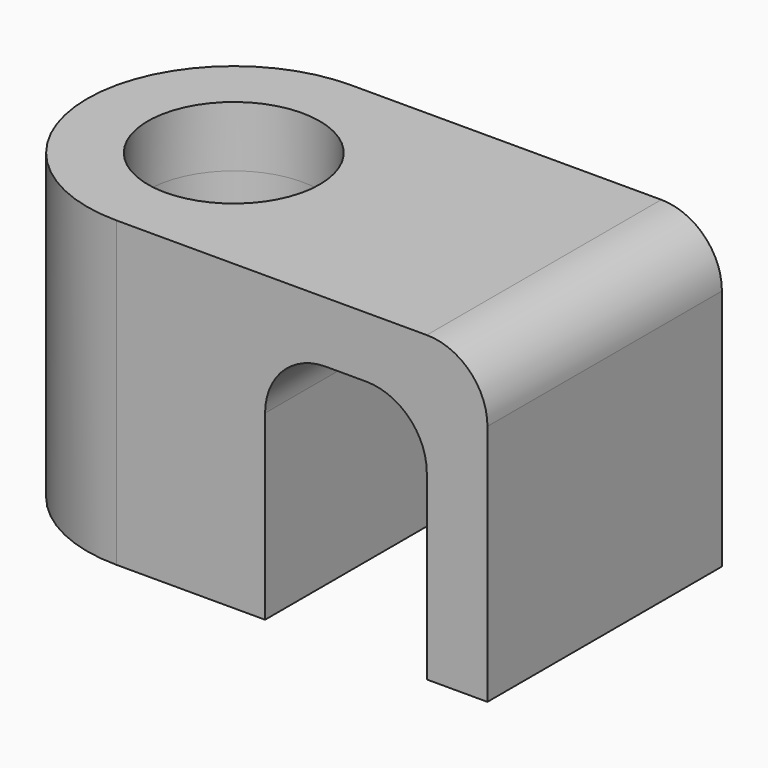
from build123d import *

# Parameters (mm, degrees)
F0_R        = 4.25
F0_W        = 8
F0_H        = 14.5
F0_W_2      = 3
F1_DEPTH    = 3
F2_DEPTH    = 12
F3_T1_DEPTH = 14.5
F3_T3_DEPTH = 29.5
F5_R        = 4.25
F6_DEPTH    = 22
F7_DEPTH    = 3
F8_T1_DEPTH = 28


# Not quite as in the source:
# - a fillet or chamfer that OpenCascade refuses, or shapes differently, is made with other operations: its cross-section is extruded or revolved along the edge and cut away or added


with BuildPart() as f1:
    # F0 (on Top) → F1 (new body)
    with BuildSketch(Plane.XY):
        with BuildLine():
            ThreePointArc((0, -7.25), (5.1265241636, -5.1265241636), (7.25, 0))
            ThreePointArc((7.25, 0), (5.1265241636, 5.1265241636), (0, 7.25))
            ThreePointArc((0, 7.25), (-7.25, 0), (0, -7.25))
        make_face()
        Circle(F0_R, mode=Mode.SUBTRACT)
        with BuildLine():
            Line((7.25, -7.25), (7.25, 0))
            ThreePointArc((7.25, 0), (5.1265241636, -5.1265241636), (0, -7.25))
            Line((0, -7.25), (7.25, -7.25))
        make_face()
        with BuildLine():
            ThreePointArc((0, 7.25), (5.1265241636, 5.1265241636), (7.25, 0))
            Line((7.25, 0), (7.25, 7.25))
            Line((7.25, 7.25), (0, 7.25))
        make_face()
        Polygon((7.25, 7.25), (7.25, 0), (7.25, -7.25), (7.35, -7.25), (7.35, 7.25), align=None)
        with Locations((11.35, 0)):
            Rectangle(F0_W, F0_H)
        with Locations((16.85, 0)):
            Rectangle(F0_W_2, F0_H)
    extrude(amount=F1_DEPTH)

    # F0 (on Top) → F2 (join)
    with BuildSketch(Plane.XY):
        with BuildLine():
            ThreePointArc((0, -7.25), (5.1265241636, -5.1265241636), (7.25, 0))
            ThreePointArc((7.25, 0), (5.1265241636, 5.1265241636), (0, 7.25))
            ThreePointArc((0, 7.25), (-7.25, 0), (0, -7.25))
        make_face()
        Circle(F0_R, mode=Mode.SUBTRACT)
        with BuildLine():
            ThreePointArc((0, 7.25), (5.1265241636, 5.1265241636), (7.25, 0))
            Line((7.25, 0), (7.25, 7.25))
            Line((7.25, 7.25), (0, 7.25))
        make_face()
        Polygon((7.25, 7.25), (7.25, 0), (7.25, -7.25), (7.35, -7.25), (7.35, 7.25), align=None)
        with Locations((16.85, 0)):
            Rectangle(F0_W_2, F0_H)
        with BuildLine():
            Line((7.25, -7.25), (7.25, 0))
            ThreePointArc((7.25, 0), (5.1265241636, -5.1265241636), (0, -7.25))
            Line((0, -7.25), (7.25, -7.25))
        make_face()
    extrude(amount=-F2_DEPTH)

    # F3: fillet of radius 3 on 3 edges, made by hand

    # F3_s2 → F3_t1 (join)
    with BuildSketch(Plane.XZ.offset(-7.25)):
        with BuildLine():
            ThreePointArc((7.35, -3), (8.2286796564, -0.8786796564), (10.35, 0))
            Line((10.35, 0), (7.35, 0))
            Line((7.35, 0), (7.35, -3))
        make_face()
        with BuildLine():
            ThreePointArc((12.35, 0), (14.4713203436, -0.8786796564), (15.35, -3))
            Line((15.35, -3), (15.35, 0))
            Line((15.35, 0), (12.35, 0))
        make_face()
    extrude(amount=F3_T1_DEPTH)

    # F3_s4 → F3_t3 (cut)
    with BuildSketch(Plane.XZ.offset(-14.75)):
        with BuildLine():
            ThreePointArc((15.35, 3), (17.4713203436, 2.1213203436), (18.35, 0))
            Line((18.35, 0), (18.35, 3))
            Line((18.35, 3), (15.35, 3))
        make_face()
    extrude(amount=F3_T3_DEPTH, mode=Mode.SUBTRACT)


with BuildPart() as f6:
    # F5 (on offset) → F6 (new body)
    with BuildSketch(Plane(origin=(0, 0, -37), x_dir=(1, 0, 0), z_dir=(0, 0, -1))):
        with BuildLine():
            Line((7.35, 7.25), (0, 7.25))
            ThreePointArc((0, 7.25), (-7.25, 0), (0, -7.25))
            Line((0, -7.25), (7.35, -7.25))
            Line((7.35, -7.25), (7.35, 7.25))
        make_face()
        Circle(F5_R, mode=Mode.SUBTRACT)
    extrude(amount=-F6_DEPTH)

    # F5 (on offset) → F7 (join)
    with BuildSketch(Plane(origin=(0, 0, -37), x_dir=(1, 0, 0), z_dir=(0, 0, -1))):
        with BuildLine():
            Line((7.35, 7.25), (0, 7.25))
            ThreePointArc((0, 7.25), (-7.25, 0), (0, -7.25))
            Line((0, -7.25), (7.35, -7.25))
            Line((7.35, -7.25), (7.35, 7.25))
        make_face()
        Circle(F5_R, mode=Mode.SUBTRACT)
        with BuildLine():
            ThreePointArc((0, -7.25), (-7.25, 0), (0, 7.25))
            Line((0, 7.25), (-37.25, 7.25))
            Line((-37.25, 7.25), (-37.25, 4))
            Line((-37.25, 4), (-22.25, 4))
            ThreePointArc((-22.25, 4), (-18.25, 0), (-22.25, -4))
            Line((-22.25, -4), (-37.25, -4))
            Line((-37.25, -4), (-37.25, -7.25))
            Line((-37.25, -7.25), (0, -7.25))
        make_face()
    extrude(amount=F7_DEPTH)

    # F8: fillet of radius 5 on 2 edges, made by hand

    # F8_s2 → F8_t1 (cut)
    with BuildSketch(Plane.XY.offset(-52.5)):
        with BuildLine():
            ThreePointArc((-32.25, -7.25), (-35.7855339059, -5.7855339059), (-37.25, -2.25))
            Line((-37.25, -2.25), (-37.25, -7.25))
            Line((-37.25, -7.25), (-32.25, -7.25))
        make_face()
        with BuildLine():
            ThreePointArc((-32.25, 7.25), (-35.7855339059, 5.7855339059), (-37.25, 2.25))
            Line((-37.25, 2.25), (-37.25, 7.25))
            Line((-37.25, 7.25), (-32.25, 7.25))
        make_face()
    extrude(amount=F8_T1_DEPTH, mode=Mode.SUBTRACT)


solid = f1.part
